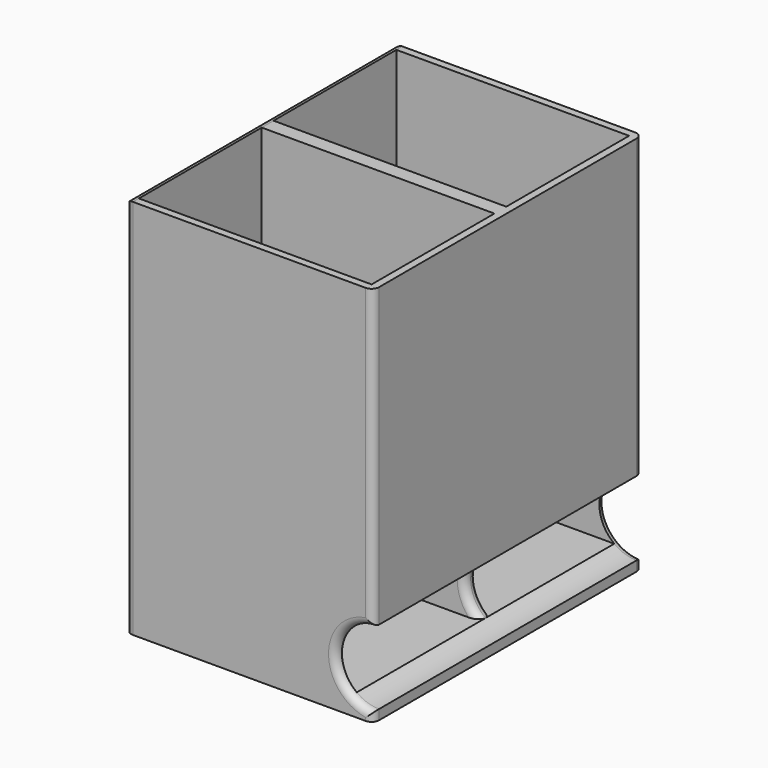
from build123d import *

# Parameters (mm, degrees)
F1_DEPTH = 34
F2_T     = -1.5
F3_DEPTH = 2
F6_R     = 1.49999


# Not quite as in the source:
# - a fillet or chamfer is up to 0.001 mm smaller than in the source, because OpenCascade refuses the exact size


with BuildPart() as f1:
    # F0 (on Front) → F1 (new body)
    with BuildSketch(Plane.XZ):
        with BuildLine():
            Line((0, 75), (-50, 75))
            Line((-50, 75), (-50, 0))
            Line((-50, 0), (0, 0))
            ThreePointArc((0, 0), (-7.5, 7.5), (0, 15))
            Line((0, 15), (0, 75))
        make_face()
    extrude(amount=F1_DEPTH)

    # F2
    f2_openings = [f1.faces().sort_by_distance(p)[0] for p in [
        (-25, -17, 75),
        (-7.5, -17, 7.5),
    ]]
    offset(amount=F2_T, openings=f2_openings)

    # F3 (add): a face of the model
    f3_faces = [f1.faces().sort_by_distance(p)[0] for p in [
        (-25, -17, 0),
    ]]
    extrude(f3_faces, amount=F3_DEPTH)


with BuildPart() as f4_1:
    # F4: instance of F1
    add(f1.part.mirror(Plane(origin=(-25.5124575843, 0, 37.1811815231), x_dir=(-1, 0, 0), z_dir=(0, 1, 0))))


with BuildPart() as f1_1:
    add(f1.part)

    # F5: union F4_1
    add(f4_1.part)

    # F6 (radius 1.5 in the source; OpenCascade refuses exactly that, so slightly less here)
    f6_edges = [f1_1.edges().sort_by_distance(p)[0] for p in [
        (0, -34, 45),
        (-50, -34, 36.5),
        (-50, 34, 36.5),
        (0, 34, -1),
        (0, -34, -1),
        (-50, 0, 75),
        (0, 34, 45),
        (-7.5, 34, 7.5),
        (-7.317473, 1.5, 9.144564),
        (-7.317473, -1.5, 9.144564),
        (-7.5, -34, 7.5),
    ]]
    fillet(f6_edges, radius=F6_R)


solid = f1_1.part
